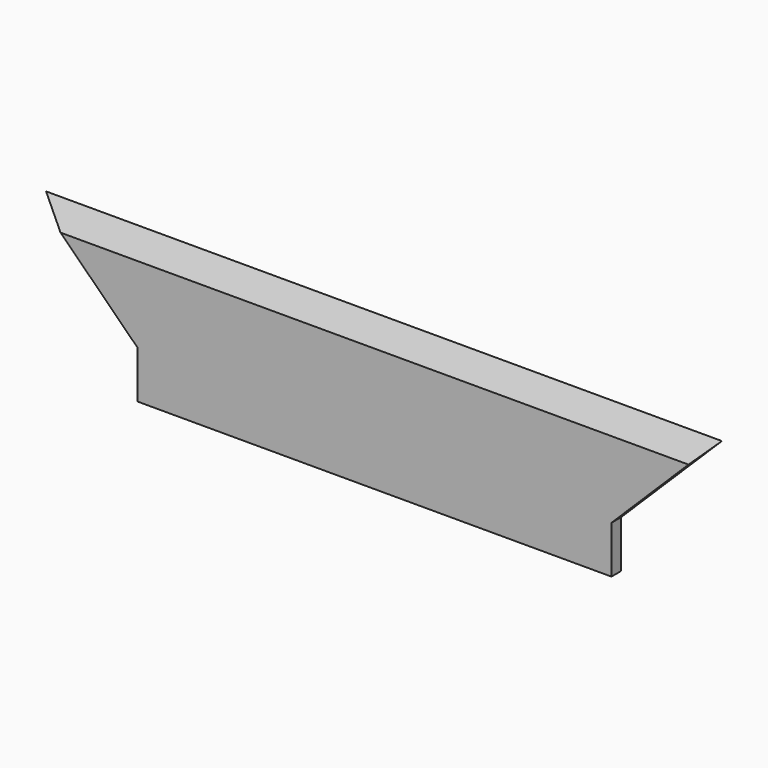
from build123d import *

# Parameters (mm, degrees)
F0_W     = 254
F0_H     = 25.4
F1_DEPTH = 6.35
F2_SIZE2 = 12.69999
F2_SIZE  = 6.34999


# Not quite as in the source:
# - a fillet or chamfer is up to 0.001 mm smaller than in the source, because OpenCascade refuses the exact size


with BuildPart() as f1:
    # F0 (on Front) → F1 (new body)
    with BuildSketch(Plane.XZ):
        with Locations((127, 12.7)):
            Rectangle(F0_W, F0_H)
        Polygon((-54.1485526787, 79.0131909403), (0, 25.4), (254, 25.4), (308.1485526787, 79.0131909403), align=None)
    extrude(amount=F1_DEPTH)

    # F2 (size 6.35 and 12.7 in the source; OpenCascade refuses exactly that, so slightly less here)
    f2_edges = [f1.edges().sort_by_distance(p)[0] for p in [
        (127, -6.35, 79.013191),
    ]]
    f2_side = f1.faces().sort_by_distance((127, -3.175, 79.013191))[0]
    chamfer(f2_edges, length=F2_SIZE, length2=F2_SIZE2, reference=f2_side)


solid = f1.part
